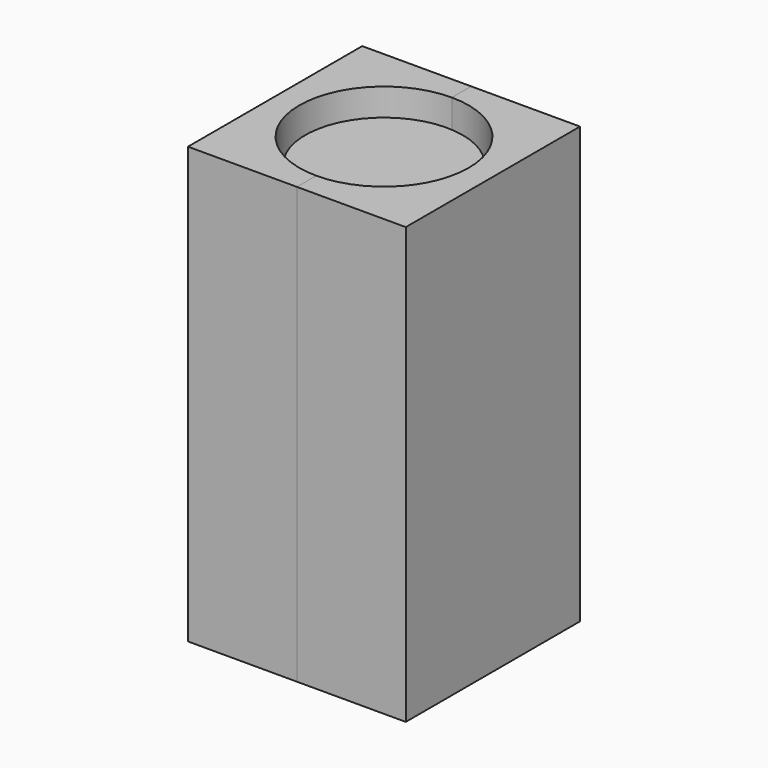
from build123d import *

# Parameters (mm, degrees)
F0_W     = 63.5
F0_H     = 114.3
F1_DEPTH = 228.6
F2_DEPTH = 228.6
F4_R     = 41.275
F5_DEPTH = 203.2
F4_R_2   = 44.45
F6_DEPTH = 215.9
F7_W     = 6.35
F7_H     = 114.3
F8_DEPTH = 228.601


with BuildPart() as f1:
    # F0 (on Top) → F1 (new body)
    with BuildSketch(Plane.XY):
        with Locations((-31.75, 0)):
            Rectangle(F0_W, F0_H)
    extrude(amount=F1_DEPTH)


with BuildPart() as f2:
    # F0 (on Top) → F2 (new body)
    with BuildSketch(Plane.XY):
        with Locations((31.75, 0)):
            Rectangle(F0_W, F0_H)
    extrude(amount=F2_DEPTH)


with BuildPart() as f5:
    # F4 (on offset) → F5 (new body)
    with BuildSketch(Plane.XY.offset(12.7)):
        Circle(F4_R)
    extrude(amount=F5_DEPTH)


with BuildPart() as f6_tool:
    # F4 (on offset) → F6 (new body, through all)
    with BuildSketch(Plane.XY.offset(12.7)):
        Circle(F4_R_2)
        Circle(F4_R, mode=Mode.SUBTRACT)
        Circle(F4_R)
    extrude(amount=F6_DEPTH)


with BuildPart() as f1_1:
    add(f1.part)

    # F6: cut by f6_tool
    add(f6_tool.part, mode=Mode.SUBTRACT)


with BuildPart() as f2_1:
    add(f2.part)

    # F6: cut by f6_tool
    add(f6_tool.part, mode=Mode.SUBTRACT)


with BuildPart() as f8_tool:
    # F7 (on Top) → F8 (new body, through all)
    with BuildSketch(Plane.XY):
        with Locations((-60.325, 0)):
            Rectangle(F7_W, F7_H)
        with Locations((60.325, 0)):
            Rectangle(F7_W, F7_H)
    extrude(amount=F8_DEPTH)


with BuildPart() as f1_2:
    add(f1_1.part)

    # F8: cut by f8_tool
    add(f8_tool.part, mode=Mode.SUBTRACT)


with BuildPart() as f2_2:
    add(f2_1.part)

    # F8: cut by f8_tool
    add(f8_tool.part, mode=Mode.SUBTRACT)


solid = Compound([f5.part, f1_2.part, f2_2.part])
